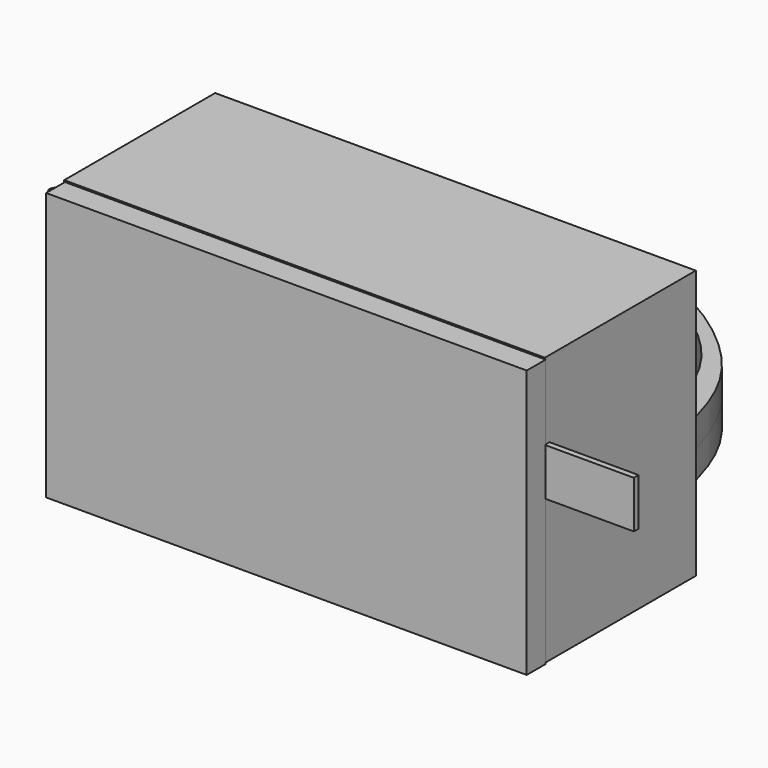
from build123d import *

# Parameters (mm, degrees)
F0_W         = 165.6168848276
F0_H         = 92.3485867679
F1_DEPTH     = 8.128
F2_W         = 65.0001764297
F2_H         = 58.7672814727
F2_H_2       = 33.835709095
F3_DEPTH     = 82.804
F4_W         = 145.6484049559
F4_H         = 80.3916100413
F5_DEPTH     = 126.492
F7_DEPTH     = 9.652
F10_DEPTH    = 7.3972418904
F11_R        = 3.6792614691
F12_W        = 10.9393596649
F12_H        = 9.4129405916
F12_W_2      = 8.9041367173
F12_H_2      = 12.2113823891
F13_DEPTH    = 3.937
F14_T1_DEPTH = 34.8129405916
F14_T3_DEPTH = 37.6046565067
F14_T5_DEPTH = 37.6113823891
F17_R        = 3.4704088756
F18_DEPTH    = 12.7
F17_R_2      = 2.9399233627
F19_W        = 34.344509244
F19_H        = 16.2818413228
F20_DEPTH    = 2.032


# Not quite as in the source:
# - a fillet or chamfer that OpenCascade refuses, or shapes differently, is made with other operations: its cross-section is extruded or revolved along the edge and cut away or added
# - the program builds the solid bodies; features that only make, move or delete a surface that nothing else refers to are left out


with BuildPart() as f1:
    # F0 (on Front) → F1 (new body)
    with BuildSketch(Plane.XZ):
        with Locations((0.2544000745, 12.0841804892)):
            Rectangle(F0_W, F0_H)
    extrude(amount=F1_DEPTH)

    # F2 (on Right) → F3 (join, symmetric)
    with BuildSketch(Plane.YZ):
        with Locations((32.5000882149, 29.3836407363)):
            Rectangle(F2_W, F2_H)
        with Locations((32.5000882149, -16.9178545475)):
            Rectangle(F2_W, F2_H_2)
    extrude(amount=F3_DEPTH, both=True)

    # F4 (on Front) → F5 (cut)
    with BuildSketch(Plane.XZ):
        with Locations((0.191912055, 12.4657889828)):
            Rectangle(F4_W, F4_H)
    extrude(amount=-F5_DEPTH, mode=Mode.SUBTRACT)

    # F6 (on Top) → F7 (join, symmetric)
    with BuildSketch(Plane.XY):
        with BuildLine():
            add(Edge.make_bspline(
                [(-79.9747332931, 59.7409568727), (-74.759309212, 71.5402326481), (-64.1121283898, 104.8437669446), (-0.8218087411, 149.2928303601), (69.0623713402, 104.8495046273), (76.000106137, 76.6716472512), (78.8641497493, 65.1005506516)],
                knots=[0, 0, 0, 0, 0.2285913714, 0.5054588291, 0.7899145134, 1, 1, 1, 1], degree=3))
            Line((-79.9747332931, 59.7409568727), (-72.1789598465, 59.7409568727))
            add(Edge.make_bspline(
                [(-72.1789598465, 59.7409568727), (-67.4777405263, 72.5239789548), (-57.1703831688, 100.5505754042), (-1.1788929882, 141.3410376084), (62.5812635029, 105.9839202997), (68.3926515764, 74.3199638324), (71.0683837533, 59.7409568727)],
                knots=[0, 0, 0, 0, 0.226520536, 0.4966430951, 0.7682398336, 1, 1, 1, 1], degree=3))
            Line((71.0683837533, 59.7409568727), (78.8641497493, 59.7409568727))
            Line((78.8641497493, 59.7409568727), (78.8641497493, 65.1005506516))
        make_face()
    extrude(amount=F7_DEPTH, both=True)

    # F10 (add): a face of the model
    f10_faces = [f1.faces().sort_by_distance(p)[0] for p in [
        (0.191912055, 0, 12.4657889828),
    ]]
    extrude(f10_faces, amount=F10_DEPTH)

    # F11
    f11_edges = [f1.edges().sort_by_distance(p)[0] for p in [
        (0.191912, 65.000176, -27.730016),
        (0.191912, 65.000176, 52.661594),
        (-72.63229, 65.000176, 31.156797),
        (73.016115, 65.000176, 31.156797),
        (73.016115, 65.000176, -18.691008),
        (-72.63229, 65.000176, -18.691008),
    ]]
    fillet(f11_edges, radius=F11_R)

    # F12 (on Front) → F13 (join, symmetric)
    with BuildSketch(Plane.XZ):
        with Locations((-82.5518220663, 49.7359465808)):
            Rectangle(F12_W, F12_H)
        with Locations((-83.3150334656, -23.1507476419)):
            Rectangle(F12_W_2, F12_H_2)
    extrude(amount=F13_DEPTH, both=True)

    # F14: fillet of radius 5.08 on 4 edges, made by hand

    # F14_s2 → F14_t1 (cut)
    with BuildSketch(Plane.XY.offset(32.329476285)):
        with BuildLine():
            ThreePointArc((-82.9415018988, 3.937), (-86.5336043472, 2.4491024484), (-88.0215018988, -1.143))
            Line((-88.0215018988, -1.143), (-88.0215018988, 3.937))
            Line((-88.0215018988, 3.937), (-82.9415018988, 3.937))
        make_face()
        with BuildLine():
            ThreePointArc((-88.0215018988, 1.143), (-86.5336043472, -2.4491024484), (-82.9415018988, -3.937))
            Line((-82.9415018988, -3.937), (-88.0215018988, -3.937))
            Line((-88.0215018988, -3.937), (-88.0215018988, 1.143))
        make_face()
    extrude(amount=F14_T1_DEPTH, mode=Mode.SUBTRACT)

    # F14_s4 → F14_t3 (cut)
    with BuildSketch(Plane.XY.offset(-41.9530758953)):
        with BuildLine():
            ThreePointArc((-82.804, 3.937), (-86.3202989517, 2.4088773385), (-87.7671018243, -1.1416548235))
            Line((-87.7671018243, -1.1416548235), (-87.7671018243, 3.937))
            Line((-87.7671018243, 3.937), (-82.804, 3.937))
        make_face()
    extrude(amount=F14_T3_DEPTH, mode=Mode.SUBTRACT)

    # F14_s6 → F14_t5 (cut)
    with BuildSketch(Plane.XY.offset(-41.9564388365)):
        with BuildLine():
            ThreePointArc((-87.7671018243, 1.143), (-86.2792042727, -2.4491024484), (-82.6871018243, -3.937))
            Line((-82.6871018243, -3.937), (-87.7671018243, -3.937))
            Line((-87.7671018243, -3.937), (-87.7671018243, 1.143))
        make_face()
    extrude(amount=F14_T5_DEPTH, mode=Mode.SUBTRACT)

    # F17 (on Top) → F18 (join, symmetric)
    with BuildSketch(Plane.XY):
        with Locations((-62.0765909553, 10.5735119432)):
            Circle(F17_R)
    extrude(amount=F18_DEPTH, both=True)

    # F19 (on Front) → F20 (join)
    with BuildSketch(Plane.XZ):
        with Locations((96.2944850326, 24.1683619097)):
            Rectangle(F19_W, F19_H)
    extrude(amount=-F20_DEPTH)


with BuildPart() as f18:
    # F17 (on Top) → F18, piece 2 (new body, symmetric)
    with BuildSketch(Plane.XY):
        with Locations((65.5294060707, 10.5735119432)):
            Circle(F17_R_2)
    extrude(amount=F18_DEPTH, both=True)


solid = Compound([f1.part, f18.part])
